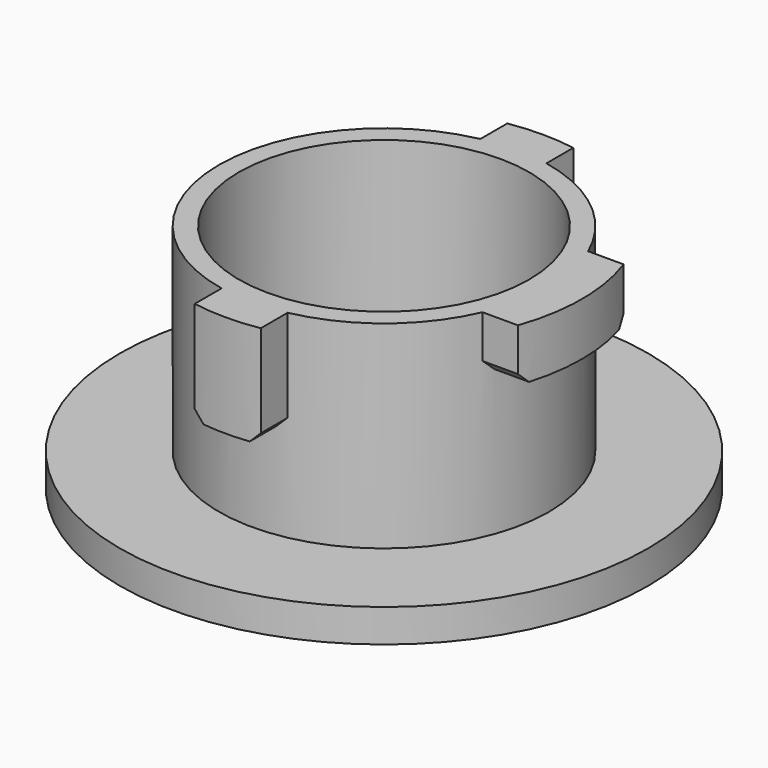
from build123d import *

# Parameters (mm, degrees)
F0_R     = 16
F0_R_2   = 8.8
F1_DEPTH = 2
F2_R     = 10
F2_R_2   = 8.8
F3_DEPTH = 12
F6_DEPTH = 6.2
F9_DEPTH = 3.2
F10_SIZE = 0.6


with BuildPart() as f1:
    # F0 (on Top) → F1 (new body)
    with BuildSketch(Plane.XY):
        Circle(F0_R)
        Circle(F0_R_2, mode=Mode.SUBTRACT)
    extrude(amount=F1_DEPTH)

    # F2 (on face) → F3 (join)
    with BuildSketch(Plane.XY.offset(2)):
        Circle(F2_R)
        Circle(F2_R_2, mode=Mode.SUBTRACT)
    extrude(amount=F3_DEPTH)

    # F5 (on offset) → F6 (join, through all)
    with BuildSketch(Plane.XY.offset(7.8)):
        with BuildLine():
            Line((-2, -9.7979589711), (-2, -11.8321595662))
            ThreePointArc((-2, -11.8321595662), (0, -12), (2, -11.8321595662))
            Line((2, -11.8321595662), (2, -9.7979589711))
            ThreePointArc((2, -9.7979589711), (0, -10), (-2, -9.7979589711))
        make_face()
        with BuildLine():
            ThreePointArc((2, 11.8321595662), (0, 12), (-2, 11.8321595662))
            Line((-2, 11.8321595662), (-2, 9.7979589711))
            ThreePointArc((-2, 9.7979589711), (0, 10), (2, 9.7979589711))
            Line((2, 9.7979589711), (2, 11.8321595662))
        make_face()
    extrude(amount=F6_DEPTH)

    # F8 (on offset) → F9 (join, through all)
    with BuildSketch(Plane.XY.offset(10.8)):
        with BuildLine():
            ThreePointArc((9.1651513899, 4), (10, 0), (9.1651513899, -4))
            Line((9.1651513899, -4), (11.313708499, -4))
            ThreePointArc((11.313708499, -4), (12, 0), (11.313708499, 4))
            Line((11.313708499, 4), (9.1651513899, 4))
        make_face()
    extrude(amount=F9_DEPTH)

    # F10
    f10_edges = [f1.edges().sort_by_distance(p)[0] for p in [
        (-8.8, 0, 0),
        (-2, 10.815059, 7.8),
        (2, 10.815059, 7.8),
        (10.23943, 4, 10.8),
        (10.23943, -4, 10.8),
        (-2, -10.815059, 7.8),
        (2, -10.815059, 7.8),
    ]]
    chamfer(f10_edges, length=F10_SIZE)


solid = f1.part
